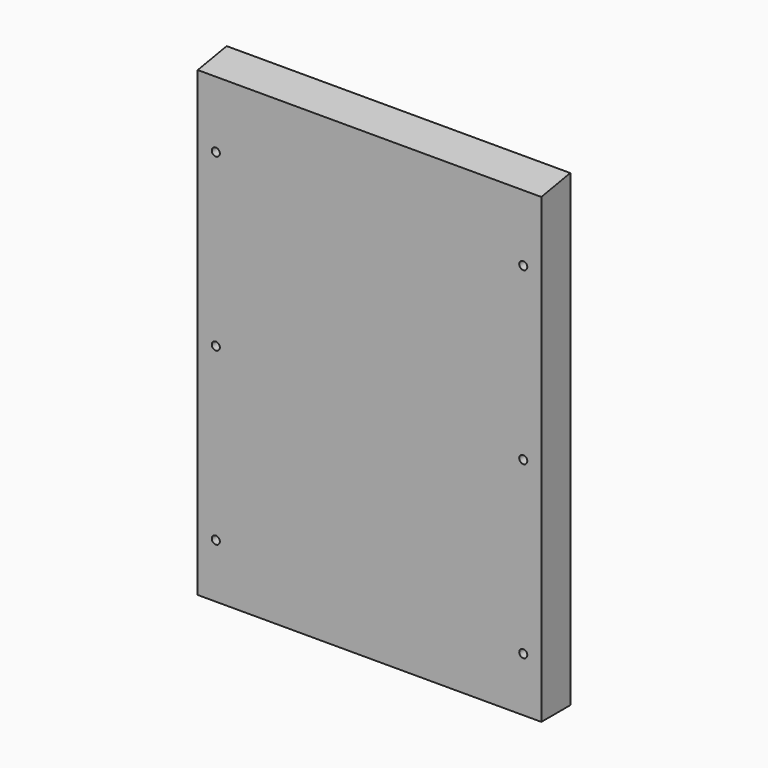
from build123d import *

# Parameters (mm, degrees)
F0_W           = 171
F0_H           = 233.17389
F1_DEPTH       = 18
F3_DEPTH       = 171.001
F5_D           = 4
F5_CSINK_D     = 8.2
F5_CSINK_ANGLE = 90


# Not quite as in the source:
# - a feature names something its author has since deleted; it is built from what else it names


with BuildPart() as f1:
    # F0 (on Front) → F1 (new body)
    with BuildSketch(Plane.XZ):
        Rectangle(F0_W, F0_H)
    extrude(amount=F1_DEPTH)

    # F2 (on face) → F3 (cut, through all)
    with BuildSketch(Plane.YZ.offset(85.5)):
        Polygon((-18, 113.4130593472), (0, 116.586945), (-18, 116.586945), align=None)
    extrude(amount=-F3_DEPTH, mode=Mode.SUBTRACT)

    # F5 (through all)
    with Locations(Plane(origin=(0, 0, 0), x_dir=(1, 0, 0), z_dir=(0, 1, 0))):
        with Locations((76.5, -80.413055), (-76.5, -80.413055), (76.5, 4.586945), (-76.5, 4.586945), (76.5, 89.586945), (-76.5, 89.586945)):
            CounterSinkHole(F5_D / 2, F5_CSINK_D / 2, counter_sink_angle=F5_CSINK_ANGLE)


solid = f1.part
